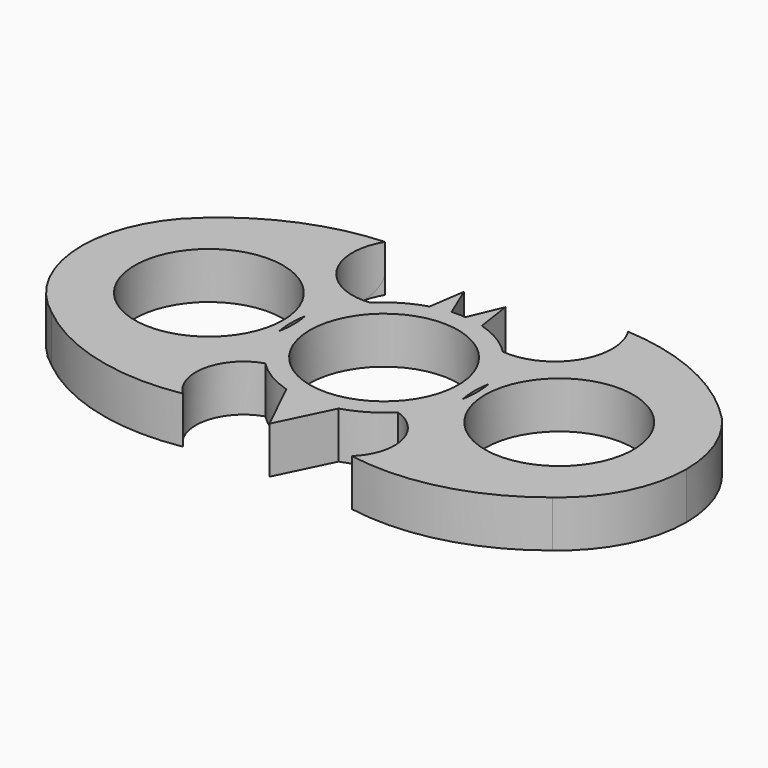
from build123d import *

# Parameters (mm, degrees)
F0_R     = 11.1125
F1_DEPTH = 6.35
F2_R     = 3.17499
F3_DEPTH = 7


# Not quite as in the source:
# - a fillet or chamfer is up to 0.001 mm smaller than in the source, because OpenCascade refuses the exact size


with BuildPart() as f1:
    # F0 (on Top) → F1 (new body)
    with BuildSketch(Plane.XY):
        with BuildLine():
            ThreePointArc((-9.9264482926, -9.8298791597), (-7.1913775024, -11.9768522417), (-4.010805007, -13.3818662075))
            ThreePointArc((-4.010805007, -13.3818662075), (-3.9641218469, -13.3957694062), (-3.9173904939, -13.4095097494))
            ThreePointArc((-3.9173904939, -13.4095097494), (0, -13.97), (3.9173904939, -13.4095097494))
            ThreePointArc((3.9173904939, -13.4095097494), (7.1495738947, -12.001853737), (9.9264482926, -9.8298791597))
            ThreePointArc((9.9264482926, -9.8298791597), (12.4120380065, -6.4111007266), (13.7613551332, -2.4054115859))
            ThreePointArc((13.7613551332, -2.4054115859), (13.5892538356, -1.2081742794), (13.5317131076, 0))
            Line((13.5317131076, 0), (11.1125, 0))
            ThreePointArc((11.1125, 0), (0, -11.1125), (-11.1125, 0))
            Line((-11.1125, 0), (-13.5317149703, 0))
            ThreePointArc((-13.5317149703, 0), (-13.589255453, -1.2081717101), (-13.7613560192, -2.4054065173))
            ThreePointArc((-13.7613560192, -2.4054065173), (-12.4120391871, -6.4110984408), (-9.9264482926, -9.8298791597))
        make_face()
        with BuildLine():
            ThreePointArc((3.9173904939, -13.4095097494), (0, -13.97), (-3.9173904939, -13.4095097494))
            Line((-3.9173904939, -13.4095097494), (0, -21.4545894414))
            Line((0, -21.4545894414), (3.9173904939, -13.4095097494))
        make_face()
        with BuildLine():
            ThreePointArc((-12.6513041413, -21.8456521056), (-14.7063688094, -15.0627697401), (-9.9264482926, -9.8298791597))
            ThreePointArc((-9.9264482926, -9.8298791597), (-12.4120391871, -6.4110984408), (-13.7613560192, -2.4054065173))
            ThreePointArc((-13.7613560192, -2.4054065173), (-13.9177412605, -1.2072192038), (-13.97, 0))
            ThreePointArc((-13.97, 0), (-13.9177412605, 1.2072192038), (-13.7613560192, 2.4054065173))
            ThreePointArc((-13.7613560192, 2.4054065173), (-12.4120395648, 6.4110977096), (-9.9264494507, 9.8298779902))
            ThreePointArc((-9.9264494507, 9.8298779902), (-18.1475057056, 13.8110021796), (-18.2071019663, 22.9450902043))
            ThreePointArc((-18.2071019663, 22.9450902043), (-30.3564318276, 19.9035068059), (-40.5314124536, 12.6009582845))
            ThreePointArc((-40.5314124536, 12.6009582845), (-45.1838875342, -2.0490994228), (-37.5057111895, -15.3650794177))
            ThreePointArc((-37.5057111895, -15.3650794177), (-25.7855371398, -21.3169777129), (-12.6513041413, -21.8456521056))
        make_face()
        with Locations((-26.2444149703, 0)):
            Circle(F0_R, mode=Mode.SUBTRACT)
        with BuildLine():
            ThreePointArc((13.7613551332, -2.4054115859), (12.4120380065, -6.4111007266), (9.9264482926, -9.8298791597))
            ThreePointArc((9.9264482926, -9.8298791597), (14.7063688094, -15.0627697401), (12.6513041413, -21.8456521056))
            ThreePointArc((12.6513041413, -21.8456521056), (25.7855371398, -21.3169777129), (37.5057111895, -15.3650794177))
            ThreePointArc((37.5057111895, -15.3650794177), (43.2360320484, -8.6132099574), (45.2944131076, 0))
            Line((45.2944131076, 0), (37.3569131076, 0))
            ThreePointArc((37.3569131076, 0), (26.2444131076, -11.1125), (15.1319131076, 0))
            Line((15.1319131076, 0), (13.97, 0))
            ThreePointArc((13.97, 0), (13.9177410382, -1.2072217669), (13.7613551332, -2.4054115859))
        make_face()
        with BuildLine():
            ThreePointArc((-13.7613560192, 2.4054065173), (-13.589255453, 1.2081717101), (-13.5317149703, 0))
            Line((-13.5317149703, 0), (-11.1125, 0))
            ThreePointArc((-11.1125, 0), (0, 11.1125), (11.1125, 0))
            Line((11.1125, 0), (13.5317131076, 0))
            ThreePointArc((13.5317131076, 0), (13.5892538356, 1.2081742794), (13.7613551332, 2.4054115859))
            ThreePointArc((13.7613551332, 2.4054115859), (12.4120383841, 6.4110999954), (9.9264494507, 9.8298779902))
            ThreePointArc((9.9264494507, 9.8298779902), (7.1495746018, 12.0018533158), (3.9173904939, 13.4095097494))
            ThreePointArc((3.9173904939, 13.4095097494), (2.4938325804, 13.7456065367), (1.0429356844, 13.9310152235))
            ThreePointArc((1.0429356844, 13.9310152235), (0, 13.97), (-1.0429356844, 13.9310152235))
            ThreePointArc((-1.0429356844, 13.9310152235), (-2.4938325804, 13.7456065367), (-3.9173904939, 13.4095097494))
            ThreePointArc((-3.9173904939, 13.4095097494), (-7.1495746018, 12.0018533158), (-9.9264494507, 9.8298779902))
            ThreePointArc((-9.9264494507, 9.8298779902), (-12.4120395648, 6.4110977096), (-13.7613560192, 2.4054065173))
        make_face()
        with BuildLine():
            ThreePointArc((13.7613551332, 2.4054115859), (13.9177410382, 1.2072217669), (13.97, 0))
            Line((13.97, 0), (15.1319131076, 0))
            ThreePointArc((15.1319131076, 0), (26.2444131076, 11.1125), (37.3569131076, 0))
            Line((37.3569131076, 0), (45.2944131076, 0))
            ThreePointArc((45.2944131076, 0), (44.0639226062, 6.7355460973), (40.5314124536, 12.6009582845))
            ThreePointArc((40.5314124536, 12.6009582845), (30.3564318276, 19.9035068059), (18.2071019663, 22.9450902043))
            ThreePointArc((18.2071019663, 22.9450902043), (18.1475057056, 13.8110021796), (9.9264494507, 9.8298779902))
            ThreePointArc((9.9264494507, 9.8298779902), (12.4120383841, 6.4110999954), (13.7613551332, 2.4054115859))
        make_face()
        with BuildLine():
            Line((-3.102583345, 18.8314262778), (-3.9173904939, 13.4095097494))
            ThreePointArc((-3.9173904939, 13.4095097494), (-2.4938325804, 13.7456065367), (-1.0429356844, 13.9310152235))
            Line((-1.0429356844, 13.9310152235), (-3.102583345, 18.8314262778))
        make_face()
        with BuildLine():
            ThreePointArc((1.0429356844, 13.9310152235), (2.4938325804, 13.7456065367), (3.9173904939, 13.4095097494))
            Line((3.9173904939, 13.4095097494), (3.102583345, 18.8314262778))
            Line((3.102583345, 18.8314262778), (1.0429356844, 13.9310152235))
        make_face()
    extrude(amount=F1_DEPTH)

    # F2 (radius 3.175 in the source; OpenCascade refuses exactly that, so slightly less here)
    f2_edges = [f1.edges().sort_by_distance(p)[0] for p in [
        (-45.183888, -2.049099, 6.35),
        (45.183888, -2.049099, 6.35),
        (45.183888, -2.049099, 0),
        (-45.183888, -2.049099, 0),
    ]]
    fillet(f2_edges, radius=F2_R)

    # F0 (on Top) → F3 (join)
    with BuildSketch(Plane.XY):
        with BuildLine():
            ThreePointArc((-9.9264482926, -9.8298791597), (-7.1913775024, -11.9768522417), (-4.010805007, -13.3818662075))
            ThreePointArc((-4.010805007, -13.3818662075), (-3.9641218469, -13.3957694062), (-3.9173904939, -13.4095097494))
            ThreePointArc((-3.9173904939, -13.4095097494), (0, -13.97), (3.9173904939, -13.4095097494))
            ThreePointArc((3.9173904939, -13.4095097494), (7.1495738947, -12.001853737), (9.9264482926, -9.8298791597))
            ThreePointArc((9.9264482926, -9.8298791597), (12.4120380065, -6.4111007266), (13.7613551332, -2.4054115859))
            ThreePointArc((13.7613551332, -2.4054115859), (13.5892538356, -1.2081742794), (13.5317131076, 0))
            Line((13.5317131076, 0), (11.1125, 0))
            ThreePointArc((11.1125, 0), (0, -11.1125), (-11.1125, 0))
            Line((-11.1125, 0), (-13.5317149703, 0))
            ThreePointArc((-13.5317149703, 0), (-13.589255453, -1.2081717101), (-13.7613560192, -2.4054065173))
            ThreePointArc((-13.7613560192, -2.4054065173), (-12.4120391871, -6.4110984408), (-9.9264482926, -9.8298791597))
        make_face()
        with BuildLine():
            ThreePointArc((3.9173904939, -13.4095097494), (0, -13.97), (-3.9173904939, -13.4095097494))
            Line((-3.9173904939, -13.4095097494), (0, -21.4545894414))
            Line((0, -21.4545894414), (3.9173904939, -13.4095097494))
        make_face()
        with BuildLine():
            ThreePointArc((-12.6513041413, -21.8456521056), (-14.7063688094, -15.0627697401), (-9.9264482926, -9.8298791597))
            ThreePointArc((-9.9264482926, -9.8298791597), (-12.4120391871, -6.4110984408), (-13.7613560192, -2.4054065173))
            ThreePointArc((-13.7613560192, -2.4054065173), (-13.9177412605, -1.2072192038), (-13.97, 0))
            ThreePointArc((-13.97, 0), (-13.9177412605, 1.2072192038), (-13.7613560192, 2.4054065173))
            ThreePointArc((-13.7613560192, 2.4054065173), (-12.4120395648, 6.4110977096), (-9.9264494507, 9.8298779902))
            ThreePointArc((-9.9264494507, 9.8298779902), (-18.1475057056, 13.8110021796), (-18.2071019663, 22.9450902043))
            ThreePointArc((-18.2071019663, 22.9450902043), (-30.3564318276, 19.9035068059), (-40.5314124536, 12.6009582845))
            ThreePointArc((-40.5314124536, 12.6009582845), (-45.1838875342, -2.0490994228), (-37.5057111895, -15.3650794177))
            ThreePointArc((-37.5057111895, -15.3650794177), (-25.7855371398, -21.3169777129), (-12.6513041413, -21.8456521056))
        make_face()
        with Locations((-26.2444149703, 0)):
            Circle(F0_R, mode=Mode.SUBTRACT)
        with BuildLine():
            ThreePointArc((13.7613551332, -2.4054115859), (12.4120380065, -6.4111007266), (9.9264482926, -9.8298791597))
            ThreePointArc((9.9264482926, -9.8298791597), (14.7063688094, -15.0627697401), (12.6513041413, -21.8456521056))
            ThreePointArc((12.6513041413, -21.8456521056), (25.7855371398, -21.3169777129), (37.5057111895, -15.3650794177))
            ThreePointArc((37.5057111895, -15.3650794177), (43.2360320484, -8.6132099574), (45.2944131076, 0))
            Line((45.2944131076, 0), (37.3569131076, 0))
            ThreePointArc((37.3569131076, 0), (26.2444131076, -11.1125), (15.1319131076, 0))
            Line((15.1319131076, 0), (13.97, 0))
            ThreePointArc((13.97, 0), (13.9177410382, -1.2072217669), (13.7613551332, -2.4054115859))
        make_face()
        with BuildLine():
            ThreePointArc((-13.7613560192, 2.4054065173), (-13.589255453, 1.2081717101), (-13.5317149703, 0))
            Line((-13.5317149703, 0), (-11.1125, 0))
            ThreePointArc((-11.1125, 0), (0, 11.1125), (11.1125, 0))
            Line((11.1125, 0), (13.5317131076, 0))
            ThreePointArc((13.5317131076, 0), (13.5892538356, 1.2081742794), (13.7613551332, 2.4054115859))
            ThreePointArc((13.7613551332, 2.4054115859), (12.4120383841, 6.4110999954), (9.9264494507, 9.8298779902))
            ThreePointArc((9.9264494507, 9.8298779902), (7.1495746018, 12.0018533158), (3.9173904939, 13.4095097494))
            ThreePointArc((3.9173904939, 13.4095097494), (2.4938325804, 13.7456065367), (1.0429356844, 13.9310152235))
            ThreePointArc((1.0429356844, 13.9310152235), (0, 13.97), (-1.0429356844, 13.9310152235))
            ThreePointArc((-1.0429356844, 13.9310152235), (-2.4938325804, 13.7456065367), (-3.9173904939, 13.4095097494))
            ThreePointArc((-3.9173904939, 13.4095097494), (-7.1495746018, 12.0018533158), (-9.9264494507, 9.8298779902))
            ThreePointArc((-9.9264494507, 9.8298779902), (-12.4120395648, 6.4110977096), (-13.7613560192, 2.4054065173))
        make_face()
        with BuildLine():
            ThreePointArc((13.7613551332, 2.4054115859), (13.9177410382, 1.2072217669), (13.97, 0))
            Line((13.97, 0), (15.1319131076, 0))
            ThreePointArc((15.1319131076, 0), (26.2444131076, 11.1125), (37.3569131076, 0))
            Line((37.3569131076, 0), (45.2944131076, 0))
            ThreePointArc((45.2944131076, 0), (44.0639226062, 6.7355460973), (40.5314124536, 12.6009582845))
            ThreePointArc((40.5314124536, 12.6009582845), (30.3564318276, 19.9035068059), (18.2071019663, 22.9450902043))
            ThreePointArc((18.2071019663, 22.9450902043), (18.1475057056, 13.8110021796), (9.9264494507, 9.8298779902))
            ThreePointArc((9.9264494507, 9.8298779902), (12.4120383841, 6.4110999954), (13.7613551332, 2.4054115859))
        make_face()
        with BuildLine():
            Line((-3.102583345, 18.8314262778), (-3.9173904939, 13.4095097494))
            ThreePointArc((-3.9173904939, 13.4095097494), (-2.4938325804, 13.7456065367), (-1.0429356844, 13.9310152235))
            Line((-1.0429356844, 13.9310152235), (-3.102583345, 18.8314262778))
        make_face()
        with BuildLine():
            ThreePointArc((1.0429356844, 13.9310152235), (2.4938325804, 13.7456065367), (3.9173904939, 13.4095097494))
            Line((3.9173904939, 13.4095097494), (3.102583345, 18.8314262778))
            Line((3.102583345, 18.8314262778), (1.0429356844, 13.9310152235))
        make_face()
    extrude(amount=F3_DEPTH)


solid = f1.part
